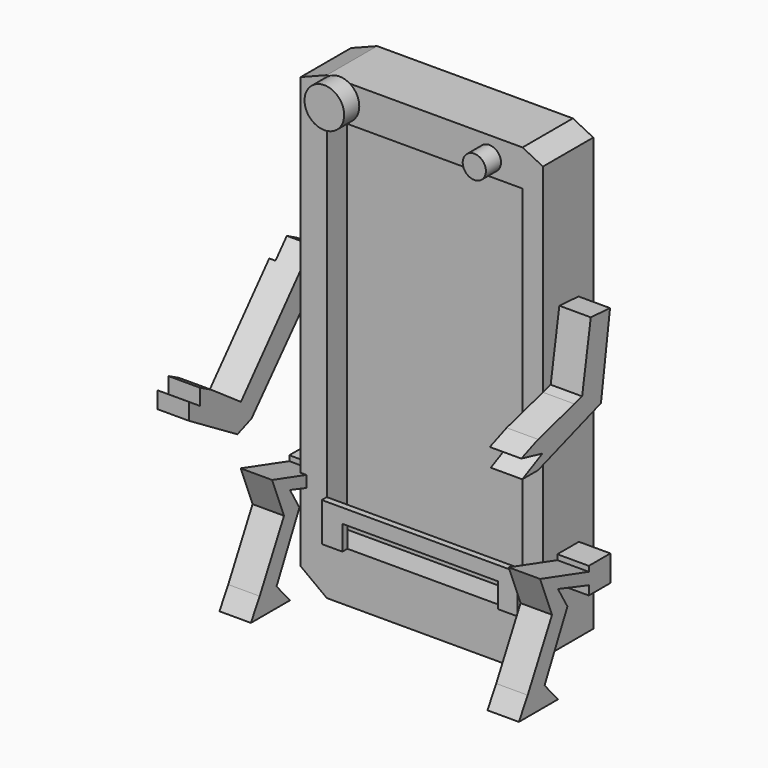
from build123d import *

# Parameters (mm, degrees)
F0_W      = 79
F0_H      = 150.9931944311
F1_DEPTH  = 15.24
F0_W_2    = 8.242815733
F0_H_2    = 14.6122574806
F0_W_3    = 10.5468220115
F2_DEPTH  = 25.4
F3_W      = 8.3270930648
F3_H      = 9.9045075476
F4_DEPTH  = 2.54
F5_R      = 8
F5_R_2    = 4.6759862525
F6_DEPTH  = 7.62
F8_DEPTH  = 10.16
F10_DEPTH = 12.7
F11_DEPTH = 12.7
F13_DEPTH = 12.7


# Not quite as in the source:
# - a pattern or mirror of a feature is missing from the dataset's text; its kind, count and spacing are read off the source's solid
# - a feature names something its author has since deleted; it is built from what else it names


with BuildPart() as f1:
    # F0 (on Front) → F1 (new body)
    with BuildSketch(Plane.XZ):
        with Locations((-116.1688212752, 21.4886832982)):
            Rectangle(F0_W, F0_H)
    extrude(amount=F1_DEPTH)

    # F0 (on Front) → F2 (join)
    with BuildSketch(Plane.XZ):
        with Locations((-72.5474134088, 21.4886832982)):
            Rectangle(F0_W_2, F0_H)
        with Locations((-116.1688212752, 104.2914092541)):
            Rectangle(F0_W, F0_H_2)
        Polygon((-76.6688212752, 111.5975379944), (-76.6688212752, 96.9852805138), (-68.4260055423, 96.9852805138), (-68.4260055423, 107.4761226773), align=None)
        Polygon((-77.7368583679, -74.2402523756), (-76.6688212752, -54.0079139173), (-155.6688212752, -54.0079139173), (-155.6688212752, -74.2402523756), align=None)
        Polygon((-68.4260055423, -54.0079139173), (-76.6688212752, -54.0079139173), (-77.7368583679, -74.2402523756), (-68.4260055423, -67.1214684844), align=None)
        with Locations((-160.942232281, 21.4886832982)):
            Rectangle(F0_W_3, F0_H)
        Polygon((-166.2156432867, 96.9852805138), (-155.6688212752, 96.9852805138), (-155.6688212752, 111.5975379944), (-166.2156432867, 107.4761226773), align=None)
        Polygon((-155.6688212752, -74.2402523756), (-155.6688212752, -54.0079139173), (-166.2156432867, -54.0079139173), (-166.2156432867, -66.3721188903), align=None)
    extrude(amount=F2_DEPTH)

    # F5 (on face) → F6 (join)
    with BuildSketch(Plane.XZ.offset(25.4)):
        with Locations((-150.5664885044, 104.7975379944)):
            Circle(F5_R)
        with Locations((-90.0309309363, 103.4603789449)):
            Circle(F5_R_2)
    extrude(amount=F6_DEPTH)

    # F7 (on face) → F8 (join)
    with BuildSketch(Plane(origin=(-166.2156432867, 0, 0), x_dir=(0, -1, 0), z_dir=(-1, 0, 0))):
        Polygon((12.5508932397, 38.3876636624), (25.4, 23.9966639606), (25.4, 38.9068748126), (19.6947995573, 45.4485118389), (14.391691424, 42.5712950528), align=None)
    extrude(amount=F8_DEPTH)

    # F9 (on face) → F10 (join)
    with BuildSketch(Plane.YZ.offset(-68.4260055423)):
        Polygon((-25.4, -37.796987619), (-25.4, -33.1461169376), (-42.7074283361, -27.9086306691), (-36.6851389408, -43.0811978877), (-48.9648841321, -66.6637793183), (-53.3993802965, -74.3656232953), (-33.6898453534, -74.3656232953), (-40.4587760568, -66.6637793183), (-28.9117768407, -43.3081761003), (-33.6898453534, -35.1456440985), align=None)
        Polygon((-18.1280039251, -40.1227921247), (-18.1280039251, -35.3467315435), (-25.4, -33.1461169376), (-25.4, -37.796987619), align=None)
        Polygon((-7.2505627759, -33.2361012697), (-18.1280039251, -33.2361012697), (-18.1280039251, -35.3467315435), (-18.1280039251, -40.1227921247), (-18.1280039251, -43.778847903), (-7.2505627759, -43.778847903), align=None)
    f10 = extrude(amount=F10_DEPTH)

    # F10_copies: F10 across plane
    add(f10.mirror(Plane(origin=(-116.168821, 0, 0), x_dir=(0, 0, -1), z_dir=(-1, 0, 0))))

    # F7 (on face) → F11 (join)
    with BuildSketch(Plane(origin=(-166.2156432867, 0, 0), x_dir=(0, -1, 0), z_dir=(-1, 0, 0))):
        Polygon((25.4, 23.9966639606), (50.2035729587, -3.7833380047), (57.3032200336, -6.5071620047), (81.7048251629, 8.1935711205), (81.7048251629, 14.9255720899), (76.265707612, 11.3043896854), (76.265707612, 17.763774842), (70.8431079984, 14.9255720899), (55.5642731488, 4.3202326633), (25.4, 38.9068748126), align=None)
    extrude(amount=F11_DEPTH)

    # F12 (on face) → F13 (join)
    with BuildSketch(Plane.YZ.offset(-68.4260055423)):
        Polygon((-25.4, 17.4681073426), (-25.4, 27.2602735729), (-43.7104962766, 22.0907106996), (-52.2158779204, 18.7307391316), (-41.5477119386, 16.1824021488), (-51.7014451325, 11.1562022939), (-43.7104962766, 11.1562022939), align=None)
        Polygon((-7.4211359024, 54.0121272206), (-17.1320363879, 54.6712055802), (-21.4885137975, 28.3645950258), (-25.4, 27.2602735729), (-25.4, 17.4681073426), (-11.9900768623, 22.0907106996), align=None)
    extrude(amount=F13_DEPTH)


with BuildPart() as f4:
    # F3 (on face) → F4 (new body)
    with BuildSketch(Plane.XZ.offset(25.4)):
        Polygon((-76.6688212752, -44.1034063697), (-76.6688212752, -38.3540131152), (-155.6688212752, -38.3540131152), (-155.6688212752, -44.1034063697), (-147.3417282104, -44.1034063697), (-84.5337882638, -44.1034063697), align=None)
        Polygon((-76.6688212752, -54.0079139173), (-76.6688212752, -44.1034063697), (-84.5337882638, -44.1034063697), (-84.5337882638, -54.0079139173), (-81.2943726778, -54.0079139173), align=None)
        with Locations((-151.5052747428, -49.0556601435)):
            Rectangle(F3_W, F3_H)
    extrude(amount=F4_DEPTH)


solid = Compound([f1.part, f4.part])
